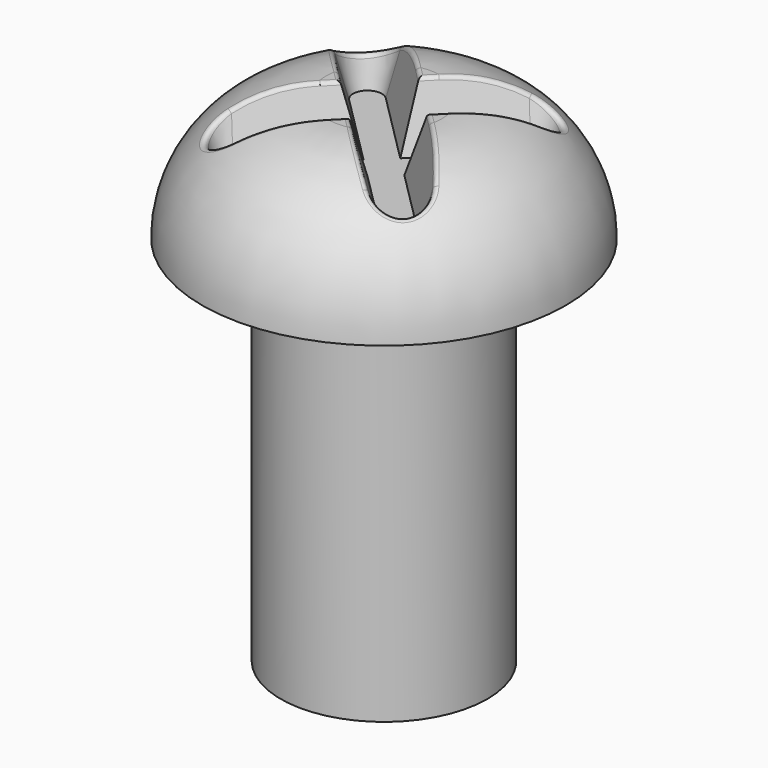
from build123d import *

# Parameters (mm, degrees)
F0_R     = 2.5
F1_DEPTH = 9
F2_R     = 4.4
F2_R_2   = 2.5
F3_DEPTH = 3
F4_R     = 2.99999
F6_DEPTH = 1.5
F6_TAPER = 15
F7_R     = 0.1


# Not quite as in the source:
# - a fillet or chamfer is up to 0.001 mm smaller than in the source, because OpenCascade refuses the exact size


with BuildPart() as f1:
    # F0 (on Top) → F1 (new body)
    with BuildSketch(Plane.XY):
        Circle(F0_R)
    extrude(amount=F1_DEPTH)

    # F2 (on face) → F3 (join)
    with BuildSketch(Plane.XY.offset(9)):
        Circle(F2_R)
        Circle(F2_R_2, mode=Mode.SUBTRACT)
        Circle(F2_R_2)
    extrude(amount=F3_DEPTH)

    # F4 (radius 3 in the source; OpenCascade refuses exactly that, so slightly less here)
    f4_edges = [f1.edges().sort_by_distance(p)[0] for p in [
        (-4.4, 0, 12),
    ]]
    fillet(f4_edges, radius=F4_R)

    # F5 (on face) → F6 (cut)
    with BuildSketch(Plane.XY.offset(12)):
        Polygon((-1.0606601718, 0), (-0.5303300859, -0.5303300859), (0, 0), (-0.5303300859, 0.5303300859), align=None)
        with BuildLine():
            Line((0, -1.0606601718), (-0.5303300859, -0.5303300859))
            Line((-0.5303300859, -0.5303300859), (-1.0606601718, 0))
            Line((-1.0606601718, 0), (-2.5303300859, -1.4696699141))
            ThreePointArc((-2.5303300859, -1.4696699141), (-2.5303300859, -2.5303300859), (-1.4696699141, -2.5303300859))
            Line((-1.4696699141, -2.5303300859), (0, -1.0606601718))
        make_face()
        Polygon((0, 0), (-0.5303300859, -0.5303300859), (0, -1.0606601718), (0.5303300859, -0.5303300859), align=None)
        Polygon((-0.5303300859, 0.5303300859), (0, 0), (0.5303300859, 0.5303300859), (0, 1.0606601718), align=None)
        Polygon((0.5303300859, 0.5303300859), (0, 0), (0.5303300859, -0.5303300859), (1.0606601718, 0), align=None)
        with BuildLine():
            Line((-2.5303300859, 1.4696699141), (-1.0606601718, 0))
            Line((-1.0606601718, 0), (-0.5303300859, 0.5303300859))
            Line((-0.5303300859, 0.5303300859), (0, 1.0606601718))
            Line((0, 1.0606601718), (-1.4696699141, 2.5303300859))
            ThreePointArc((-1.4696699141, 2.5303300859), (-2.5303300859, 2.5303300859), (-2.5303300859, 1.4696699141))
        make_face()
        with BuildLine():
            Line((0.5303300859, -0.5303300859), (0, -1.0606601718))
            Line((0, -1.0606601718), (1.4696699141, -2.5303300859))
            ThreePointArc((1.4696699141, -2.5303300859), (2.5303300859, -2.5303300859), (2.5303300859, -1.4696699141))
            Line((2.5303300859, -1.4696699141), (1.0606601718, 0))
            Line((1.0606601718, 0), (0.5303300859, -0.5303300859))
        make_face()
        with BuildLine():
            Line((0, 1.0606601718), (0.5303300859, 0.5303300859))
            Line((0.5303300859, 0.5303300859), (1.0606601718, 0))
            Line((1.0606601718, 0), (2.5303300859, 1.4696699141))
            ThreePointArc((2.5303300859, 1.4696699141), (2.5303300859, 2.5303300859), (1.4696699141, 2.5303300859))
            Line((1.4696699141, 2.5303300859), (0, 1.0606601718))
        make_face()
    extrude(amount=-F6_DEPTH, taper=F6_TAPER, mode=Mode.SUBTRACT)

    # F7
    f7_edges = [f1.edges().sort_by_distance(p)[0] for p in [
        (0.925446, -1.949244, 11.902721),
        (1.949244, 0.925446, 11.902721),
        (0.925446, 1.949244, 11.902721),
        (-0.925446, 1.949244, 11.902721),
        (-1.949244, -0.925446, 11.902721),
    ]]
    fillet(f7_edges, radius=F7_R)


solid = f1.part
